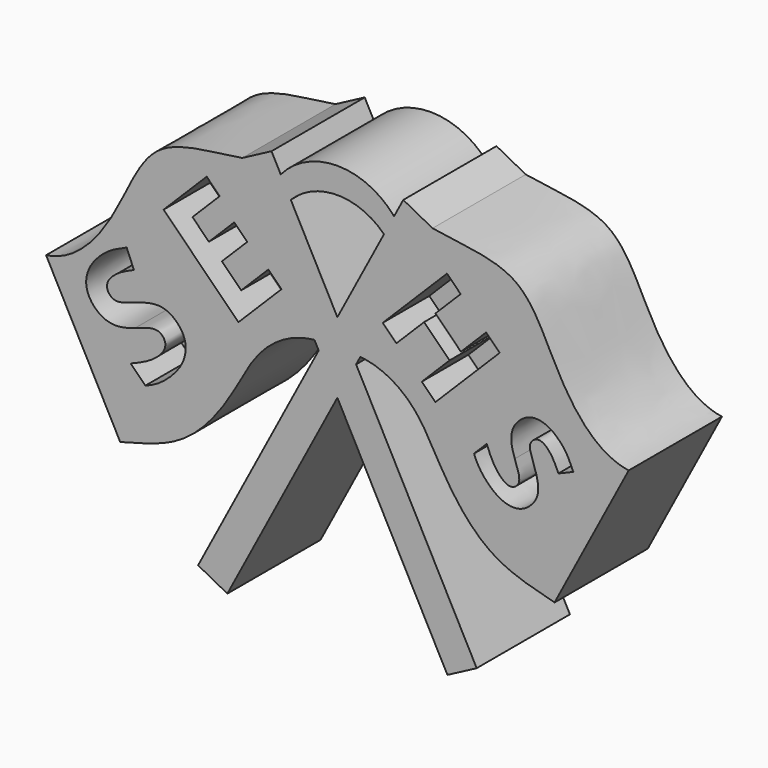
from build123d import *

# Parameters (mm, degrees)
F1_DEPTH       = 25.4
F3_DEPTH       = 25.4
F5_TEXT_SIZE   = 32.2942445226
F5_TEXT_SIZE_2 = 27.7622718845
F6_DEPTH       = 12.7


# Not quite as in the source:
# - Text() gives the source's letters only with a copy of the font that has no kerning and outlines rounded to 1/6400 em; it was checked with that copy


with BuildPart() as f1:
    # F0 (on Front) → F1 (new body)
    with BuildSketch(Plane.XZ):
        with BuildLine():
            add(Edge.make_bspline(
                [(20.7398820823, 46.1302062889), (27.1690705455, 44.9723398764), (41.0367077687, 44.9339116537), (47.4082194271, 26.340414656), (56.7587509703, 14.5510277188), (63.5, 13.5659137906)],
                knots=[0, 0, 0, 0, 0.3301882054, 0.6557983726, 1, 1, 1, 1], degree=3))
            Line((20.7398820823, 46.1302062889), (5.0048471882, 16.3460285041))
            add(Edge.make_bspline(
                [(47.3363657895, -17.0295413967), (42.4833452003, -15.7418952245), (32.6275878457, -13.4809446308), (22.5857256633, -0.2086289701), (17.7482722152, 10.756866958), (10.0349305958, 15.8277671298), (5.0048471882, 16.3460285041)],
                knots=[0, 0, 0, 0, 0.2578968635, 0.5239597623, 0.7555526652, 1, 1, 1, 1], degree=3))
            Line((47.3363657895, -17.0295413967), (63.5, 13.5659137906))
        make_face()
        Polygon((5.0048471882, 16.3460285041), (20.7398820823, 46.1302062889), (14.3619198834, 49.4996952329), (0, 22.3146284049), (4.0790346455, 14.5935973496), align=None)
        Polygon((30.3644715269, -35.1609872758), (4.0790346455, 14.5935973496), (0, 6.8725662944), (23.986509328, -38.5304762199), align=None)
        Polygon((0, 6.8725662944), (4.0790346455, 14.5935973496), (0, 22.3146284049), (-4.0790346455, 14.5935973496), align=None)
        Polygon((-4.0790346455, 14.5935973496), (0, 22.3146284049), (-14.3619198834, 49.4996952329), (-20.7398820823, 46.1302062889), (-5.0048471882, 16.3460285041), align=None)
        Polygon((-23.986509328, -38.5304762199), (0, 6.8725662944), (-4.0790346455, 14.5935973496), (-30.3644715269, -35.1609872758), align=None)
        with BuildLine():
            Line((-5.0048471882, 16.3460285041), (-20.7398820823, 46.1302062889))
            add(Edge.make_bspline(
                [(-20.7398820823, 46.1302062889), (-27.1690705455, 44.9723398764), (-41.0367077687, 44.9339116537), (-47.4082194271, 26.340414656), (-56.7587509703, 14.5510277188), (-63.5, 13.5659137906)],
                knots=[0, 0, 0, 0, 0.3301882054, 0.6557983726, 1, 1, 1, 1], degree=3))
            Line((-63.5, 13.5659137906), (-47.3363657895, -17.0295413967))
            add(Edge.make_bspline(
                [(-47.3363657895, -17.0295413967), (-42.4833452003, -15.7418952245), (-32.6275878457, -13.4809446308), (-22.5857256633, -0.2086289701), (-17.7482722152, 10.756866958), (-10.0349305958, 15.8277671298), (-5.0048471882, 16.3460285041)],
                knots=[0, 0, 0, 0, 0.2578968635, 0.5239597623, 0.7555526652, 1, 1, 1, 1], degree=3))
        make_face()
    extrude(amount=F1_DEPTH)

    # F2 (on Front) → F3 (join)
    with BuildSketch(Plane.XZ):
        with BuildLine():
            Line((12.4062707611, 38.6245631295), (14.4041060465, 42.6913709545))
            ThreePointArc((14.4041060465, 42.6913709545), (-0.4541881924, 51.3772484783), (-14.804922169, 41.8762058839))
            Line((-14.804922169, 41.8762058839), (-12.7355261447, 38.0265964086))
            ThreePointArc((-12.7355261447, 38.0265964086), (-0.3413111875, 45.754321889), (12.4062707611, 38.6245631295))
        make_face()
    extrude(amount=F3_DEPTH)

    # F5 (on offset) → F6 (cut)
    with BuildSketch(Plane.XZ.offset(25.4)):
        with Locations(Location((-42.1402398004, -6.2257256855), (0, 0, 45))):
            Text('S E', F5_TEXT_SIZE, font='Open Sans', font_style=FontStyle.BOLD, text_align=(TextAlign.LEFT, TextAlign.BOTTOM))
        with Locations(Location((8.1131019103, 26.2124841623), (0, 0, -45))):
            Text('H S', F5_TEXT_SIZE_2, font='Open Sans', font_style=FontStyle.BOLD, text_align=(TextAlign.LEFT, TextAlign.BOTTOM))
    extrude(amount=-F6_DEPTH, mode=Mode.SUBTRACT)


solid = f1.part
